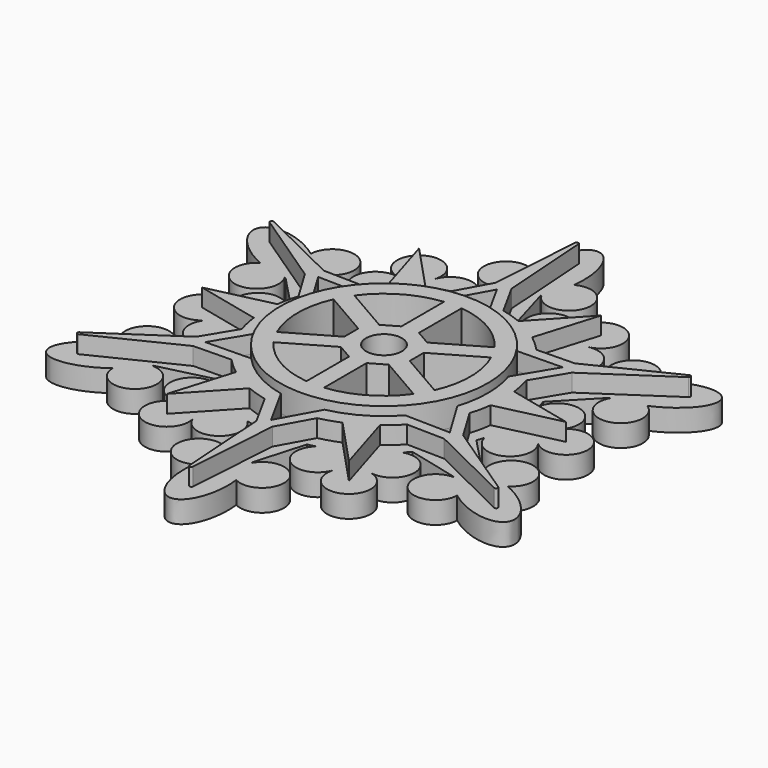
from build123d import *
from build123d import SkipClean  # not in build123d's __all__

# Parameters (mm, degrees)
F1_DEPTH      = 0.5
F3_DEPTH      = 0.4
F4_R          = 2.3683701977
F5_DEPTH      = 0.2
F5_DEPTH_BACK = 0.9
F6_R          = 0.4084956612
F7_DEPTH      = 1.1
F9_DEPTH      = 0.5


with BuildPart() as f1:
    # F0 (on Top) → F1 (new body)
    with BuildSketch(Plane.XY):
        with BuildLine():
            ThreePointArc((2.1292437706, 2.1379604716), (2.784209027, 2.5873993383), (2.1788959991, 3.1017639174))
            ThreePointArc((2.1788959991, 3.1017639174), (2.3229207895, 4.0234168295), (1.5967583495, 3.4378612461))
            ThreePointArc((1.5967583495, 3.4378612461), (0.8486490432, 3.704895416), (0.7869061954, 2.912959432))
            ThreePointArc((0.7869061954, 2.912959432), (0.6988064817, 2.9353404426), (0.6100725944, 2.9550576039))
            Line((0.6100725944, 2.9550576039), (0.2748547939, 4.1143940162))
            Line((0.2748547939, 4.1143940162), (0.2878654298, 4.1219057103))
            ThreePointArc((0.2878654298, 4.1219057103), (1.2019532573, 4.2356459456), (0.4832848134, 4.8118482237))
            add(Edge.make_bspline(
                [(0.4832848134, 4.8118482237), (0.6439857116, 6.079306826), (0, 6.079306826), (-0.6439857116, 6.079306826), (-0.4832848134, 4.8118482237)],
                knots=[4.4601826536, 4.4601826536, 4.4601826536, 6.2831853072, 6.2831853072, 8.1061879607, 8.1061879607, 8.1061879607], degree=2, weights=[1, 0.6125597551, 1, 0.6125597551, 1]))
            ThreePointArc((-0.4832848134, 4.8118482237), (-1.2019532573, 4.2356459456), (-0.2878654298, 4.1219057103))
            Line((-0.2878654298, 4.1219057103), (-0.2748547939, 4.1143940162))
            Line((-0.2748547939, 4.1143940162), (-0.6100725944, 2.9550576039))
            ThreePointArc((-0.6100725944, 2.9550576039), (-0.6988064817, 2.9353404426), (-0.7869061954, 2.912959432))
            ThreePointArc((-0.7869061954, 2.912959432), (-0.8486490432, 3.704895416), (-1.5967583495, 3.4378612461))
            ThreePointArc((-1.5967583495, 3.4378612461), (-2.3229207895, 4.0234168295), (-2.1788959991, 3.1017639174))
            ThreePointArc((-2.1788959991, 3.1017639174), (-2.784209027, 2.5873993383), (-2.1292437706, 2.1379604716))
            ThreePointArc((-2.1292437706, 2.1379604716), (-2.1926761512, 2.0728543867), (-2.2541186574, 2.0058671668))
            Line((-2.2541186574, 2.0058671668), (-3.4257423422, 2.2952282419))
            Line((-3.4257423422, 2.2952282419), (-3.4257423422, 2.3102516302))
            ThreePointArc((-3.4257423422, 2.3102516302), (-3.0672003617, 3.1587450278), (-3.9255403942, 2.8244610375))
            add(Edge.make_bspline(
                [(-3.9255403942, 2.8244610375), (-4.9428412929, 3.5973613989), (-5.2648341487, 3.039653413), (-5.5868270045, 2.4819454271), (-4.4088252076, 1.9873871862)],
                knots=[4.4601826536, 4.4601826536, 4.4601826536, 6.2831853072, 6.2831853072, 8.1061879607, 8.1061879607, 8.1061879607], degree=2, weights=[1, 0.6125597551, 1, 0.6125597551, 1]))
            ThreePointArc((-4.4088252076, 1.9873871862), (-4.269153619, 1.0769009178), (-3.713607772, 1.8116540801))
            Line((-3.713607772, 1.8116540801), (-3.7005971361, 1.8191657742))
            Line((-3.7005971361, 1.8191657742), (-2.8641912518, 0.9491904371))
            ThreePointArc((-2.8641912518, 0.9491904371), (-2.8914826329, 0.8624860559), (-2.916149966, 0.7749989604))
            ThreePointArc((-2.916149966, 0.7749989604), (-3.6328580702, 1.1174960777), (-3.7756543486, 0.3360973287))
            ThreePointArc((-3.7756543486, 0.3360973287), (-4.6458415791, 0), (-3.7756543486, -0.3360973287))
            ThreePointArc((-3.7756543486, -0.3360973287), (-3.6328580702, -1.1174960777), (-2.916149966, -0.7749989604))
            ThreePointArc((-2.916149966, -0.7749989604), (-2.8914826329, -0.8624860559), (-2.8641912518, -0.9491904371))
            Line((-2.8641912518, -0.9491904371), (-3.7005971361, -1.8191657742))
            Line((-3.7005971361, -1.8191657742), (-3.713607772, -1.8116540801))
            ThreePointArc((-3.713607772, -1.8116540801), (-4.269153619, -1.0769009178), (-4.4088252076, -1.9873871862))
            add(Edge.make_bspline(
                [(-4.4088252076, -1.9873871862), (-5.5868270045, -2.4819454271), (-5.2648341487, -3.039653413), (-4.9428412929, -3.5973613989), (-3.9255403942, -2.8244610375)],
                knots=[4.4601826536, 4.4601826536, 4.4601826536, 6.2831853072, 6.2831853072, 8.1061879607, 8.1061879607, 8.1061879607], degree=2, weights=[1, 0.6125597551, 1, 0.6125597551, 1]))
            ThreePointArc((-3.9255403942, -2.8244610375), (-3.0672003617, -3.1587450278), (-3.4257423422, -2.3102516302))
            Line((-3.4257423422, -2.3102516302), (-3.4257423422, -2.2952282419))
            Line((-3.4257423422, -2.2952282419), (-2.2541186574, -2.0058671668))
            ThreePointArc((-2.2541186574, -2.0058671668), (-2.1926761512, -2.0728543867), (-2.1292437706, -2.1379604716))
            ThreePointArc((-2.1292437706, -2.1379604716), (-2.784209027, -2.5873993383), (-2.1788959991, -3.1017639174))
            ThreePointArc((-2.1788959991, -3.1017639174), (-2.3229207895, -4.0234168295), (-1.5967583495, -3.4378612461))
            ThreePointArc((-1.5967583495, -3.4378612461), (-0.8486490432, -3.704895416), (-0.7869061954, -2.912959432))
            ThreePointArc((-0.7869061954, -2.912959432), (-0.6988064817, -2.9353404426), (-0.6100725944, -2.9550576039))
            Line((-0.6100725944, -2.9550576039), (-0.2748547939, -4.1143940162))
            Line((-0.2748547939, -4.1143940162), (-0.2878654298, -4.1219057103))
            ThreePointArc((-0.2878654298, -4.1219057103), (-1.2019532573, -4.2356459456), (-0.4832848134, -4.8118482237))
            add(Edge.make_bspline(
                [(-0.4832848134, -4.8118482237), (-0.6439857116, -6.079306826), (0, -6.079306826), (0.6439857116, -6.079306826), (0.4832848134, -4.8118482237)],
                knots=[4.4601826536, 4.4601826536, 4.4601826536, 6.2831853072, 6.2831853072, 8.1061879607, 8.1061879607, 8.1061879607], degree=2, weights=[1, 0.6125597551, 1, 0.6125597551, 1]))
            ThreePointArc((0.4832848134, -4.8118482237), (1.2019532573, -4.2356459456), (0.2878654298, -4.1219057103))
            Line((0.2878654298, -4.1219057103), (0.2748547939, -4.1143940162))
            Line((0.2748547939, -4.1143940162), (0.6100725944, -2.9550576039))
            ThreePointArc((0.6100725944, -2.9550576039), (0.6988064817, -2.9353404426), (0.7869061954, -2.912959432))
            ThreePointArc((0.7869061954, -2.912959432), (0.8486490432, -3.704895416), (1.5967583495, -3.4378612461))
            ThreePointArc((1.5967583495, -3.4378612461), (2.3229207895, -4.0234168295), (2.1788959991, -3.1017639174))
            ThreePointArc((2.1788959991, -3.1017639174), (2.784209027, -2.5873993383), (2.1292437706, -2.1379604716))
            ThreePointArc((2.1292437706, -2.1379604716), (2.1926761512, -2.0728543867), (2.2541186574, -2.0058671668))
            Line((2.2541186574, -2.0058671668), (3.4257423422, -2.2952282419))
            Line((3.4257423422, -2.2952282419), (3.4257423422, -2.3102516302))
            ThreePointArc((3.4257423422, -2.3102516302), (3.0672003617, -3.1587450278), (3.9255403942, -2.8244610375))
            add(Edge.make_bspline(
                [(3.9255403942, -2.8244610375), (4.9428412929, -3.5973613989), (5.2648341487, -3.039653413), (5.5868270045, -2.4819454271), (4.4088252076, -1.9873871862)],
                knots=[4.4601826536, 4.4601826536, 4.4601826536, 6.2831853072, 6.2831853072, 8.1061879607, 8.1061879607, 8.1061879607], degree=2, weights=[1, 0.6125597551, 1, 0.6125597551, 1]))
            ThreePointArc((4.4088252076, -1.9873871862), (4.269153619, -1.0769009178), (3.713607772, -1.8116540801))
            Line((3.713607772, -1.8116540801), (3.7005971361, -1.8191657742))
            Line((3.7005971361, -1.8191657742), (2.8641912518, -0.9491904371))
            ThreePointArc((2.8641912518, -0.9491904371), (2.8914826329, -0.8624860559), (2.916149966, -0.7749989604))
            ThreePointArc((2.916149966, -0.7749989604), (3.6328580702, -1.1174960777), (3.7756543486, -0.3360973287))
            ThreePointArc((3.7756543486, -0.3360973287), (4.6458415791, 0), (3.7756543486, 0.3360973287))
            ThreePointArc((3.7756543486, 0.3360973287), (3.6328580702, 1.1174960777), (2.916149966, 0.7749989604))
            ThreePointArc((2.916149966, 0.7749989604), (2.8914826329, 0.8624860559), (2.8641912518, 0.9491904371))
            Line((2.8641912518, 0.9491904371), (3.7005971361, 1.8191657742))
            Line((3.7005971361, 1.8191657742), (3.713607772, 1.8116540801))
            ThreePointArc((3.713607772, 1.8116540801), (4.269153619, 1.0769009178), (4.4088252076, 1.9873871862))
            add(Edge.make_bspline(
                [(4.4088252076, 1.9873871862), (5.5868270045, 2.4819454271), (5.2648341487, 3.039653413), (4.9428412929, 3.5973613989), (3.9255403942, 2.8244610375)],
                knots=[4.4601826536, 4.4601826536, 4.4601826536, 6.2831853072, 6.2831853072, 8.1061879607, 8.1061879607, 8.1061879607], degree=2, weights=[1, 0.6125597551, 1, 0.6125597551, 1]))
            ThreePointArc((3.9255403942, 2.8244610375), (3.0672003617, 3.1587450278), (3.4257423422, 2.3102516302))
            Line((3.4257423422, 2.3102516302), (3.4257423422, 2.2952282419))
            Line((3.4257423422, 2.2952282419), (2.2541186574, 2.0058671668))
            ThreePointArc((2.2541186574, 2.0058671668), (2.1926761512, 2.0728543867), (2.1292437706, 2.1379604716))
        make_face()
    extrude(amount=F1_DEPTH)

    # F2 (on face) → F3 (join)
    with BuildSketch(Plane.XY.offset(0.5)):
        with BuildLine():
            Line((-0.1806932342, 3.4074762445), (-0.597129254, 2.6519753366))
            ThreePointArc((-0.597129254, 2.6519753366), (-0.8306085867, 2.5883635578), (-1.0575056858, 2.5042400557))
            ThreePointArc((-1.0575056858, 2.5042400557), (-1.3591850989, 2.3541776481), (-1.6399826625, 2.1679468164))
            ThreePointArc((-1.6399826625, 2.1679468164), (-1.826284302, 2.0135099156), (-1.9981133847, 1.8431167716))
            Line((-1.9981133847, 1.8431167716), (-2.8606143735, 1.8602230533))
            Line((-2.8606143735, 1.8602230533), (-4.7338257783, 2.7791583452))
            ThreePointArc((-4.7338257783, 2.7791583452), (-4.7860838158, 2.7632467794), (-4.7737346173, 2.7100342085))
            Line((-4.7737346173, 2.7100342085), (-3.0413076076, 1.5472531912))
            Line((-3.0413076076, 1.5472531912), (-2.5952426387, 0.808858565))
            ThreePointArc((-2.5952426387, 0.808858565), (-2.6568928887, 0.5748536422), (-2.6974883483, 0.3362932393))
            ThreePointArc((-2.6974883483, 0.3362932393), (-2.7183701977, 0), (-2.6974883483, -0.3362932393))
            ThreePointArc((-2.6974883483, -0.3362932393), (-2.6568928887, -0.5748536422), (-2.5952426387, -0.808858565))
            Line((-2.5952426387, -0.808858565), (-3.0413076076, -1.5472531912))
            Line((-3.0413076076, -1.5472531912), (-4.7737346173, -2.7100342085))
            ThreePointArc((-4.7737346173, -2.7100342085), (-4.7860838158, -2.7632467794), (-4.7338257783, -2.7791583452))
            Line((-4.7338257783, -2.7791583452), (-2.8606143735, -1.8602230533))
            Line((-2.8606143735, -1.8602230533), (-1.9981133847, -1.8431167716))
            ThreePointArc((-1.9981133847, -1.8431167716), (-1.826284302, -2.0135099156), (-1.6399826625, -2.1679468164))
            ThreePointArc((-1.6399826625, -2.1679468164), (-1.3591850989, -2.3541776481), (-1.0575056858, -2.5042400557))
            ThreePointArc((-1.0575056858, -2.5042400557), (-0.8306085867, -2.5883635578), (-0.597129254, -2.6519753366))
            Line((-0.597129254, -2.6519753366), (-0.1806932342, -3.4074762445))
            Line((-0.1806932342, -3.4074762445), (-0.039908839, -5.4891925537))
            ThreePointArc((-0.039908839, -5.4891925537), (0, -5.5264935588), (0.039908839, -5.4891925537))
            Line((0.039908839, -5.4891925537), (0.1806932342, -3.4074762445))
            Line((0.1806932342, -3.4074762445), (0.597129254, -2.6519753366))
            ThreePointArc((0.597129254, -2.6519753366), (0.8306085867, -2.5883635578), (1.0575056858, -2.5042400557))
            ThreePointArc((1.0575056858, -2.5042400557), (1.3591850989, -2.3541776481), (1.6399826625, -2.1679468164))
            ThreePointArc((1.6399826625, -2.1679468164), (1.826284302, -2.0135099156), (1.9981133847, -1.8431167716))
            Line((1.9981133847, -1.8431167716), (2.8606143735, -1.8602230533))
            Line((2.8606143735, -1.8602230533), (4.7338257783, -2.7791583452))
            ThreePointArc((4.7338257783, -2.7791583452), (4.7860838158, -2.7632467794), (4.7737346173, -2.7100342085))
            Line((4.7737346173, -2.7100342085), (3.0413076076, -1.5472531912))
            Line((3.0413076076, -1.5472531912), (2.5952426387, -0.808858565))
            ThreePointArc((2.5952426387, -0.808858565), (2.6568928887, -0.5748536422), (2.6974883483, -0.3362932393))
            ThreePointArc((2.6974883483, -0.3362932393), (2.7183701977, 0), (2.6974883483, 0.3362932393))
            ThreePointArc((2.6974883483, 0.3362932393), (2.6568928887, 0.5748536422), (2.5952426387, 0.808858565))
            Line((2.5952426387, 0.808858565), (3.0413076076, 1.5472531912))
            Line((3.0413076076, 1.5472531912), (4.7737346173, 2.7100342085))
            ThreePointArc((4.7737346173, 2.7100342085), (4.7860838158, 2.7632467794), (4.7338257783, 2.7791583452))
            Line((4.7338257783, 2.7791583452), (2.8606143735, 1.8602230533))
            Line((2.8606143735, 1.8602230533), (1.9981133847, 1.8431167716))
            ThreePointArc((1.9981133847, 1.8431167716), (1.826284302, 2.0135099156), (1.6399826625, 2.1679468164))
            ThreePointArc((1.6399826625, 2.1679468164), (1.3591850989, 2.3541776481), (1.0575056858, 2.5042400557))
            ThreePointArc((1.0575056858, 2.5042400557), (0.8306085867, 2.5883635578), (0.597129254, 2.6519753366))
            Line((0.597129254, 2.6519753366), (0.1806932342, 3.4074762445))
            Line((0.1806932342, 3.4074762445), (0.039908839, 5.4891925537))
            ThreePointArc((0.039908839, 5.4891925537), (0, 5.5264935588), (-0.039908839, 5.4891925537))
            Line((-0.039908839, 5.4891925537), (-0.1806932342, 3.4074762445))
        make_face()
        Polygon((-2.1979116775, -0.6346252141), (-1.6485573961, -1.5861347409), (-2.786351891, -1.6087010143), align=None, mode=Mode.SUBTRACT)
        Polygon((-0.5493542814, -2.220759955), (0.5493542814, -2.220759955), (0, -3.2174020287), align=None, mode=Mode.SUBTRACT)
        Polygon((1.6485573961, -1.5861347409), (2.1979116775, -0.6346252141), (2.786351891, -1.6087010143), align=None, mode=Mode.SUBTRACT)
        Polygon((-1.6485573961, 1.5861347409), (-2.1979116775, 0.6346252141), (-2.786351891, 1.6087010143), align=None, mode=Mode.SUBTRACT)
        Polygon((2.1979116775, 0.6346252141), (1.6485573961, 1.5861347409), (2.786351891, 1.6087010143), align=None, mode=Mode.SUBTRACT)
        Polygon((-0.5493542814, 2.220759955), (0, 3.2174020287), (0.5493542814, 2.220759955), align=None, mode=Mode.SUBTRACT)
        with BuildLine():
            ThreePointArc((-1.6399826625, 2.1679468164), (-1.3591850989, 2.3541776481), (-1.0575056858, 2.5042400557))
            Line((-1.0575056858, 2.5042400557), (-2.0729207895, 3.5904041276))
            Line((-2.0729207895, 3.5904041276), (-1.6399826625, 2.1679468164))
        make_face()
        with BuildLine():
            Line((2.0729207895, 3.5904041276), (1.0575056858, 2.5042400557))
            ThreePointArc((1.0575056858, 2.5042400557), (1.3591850989, 2.3541776481), (1.6399826625, 2.1679468164))
            Line((1.6399826625, 2.1679468164), (2.0729207895, 3.5904041276))
        make_face()
        with BuildLine():
            ThreePointArc((-2.6974883483, -0.3362932393), (-2.7183701977, 0), (-2.6974883483, 0.3362932393))
            Line((-2.6974883483, 0.3362932393), (-4.1458415791, 0))
            Line((-4.1458415791, 0), (-2.6974883483, -0.3362932393))
        make_face()
        with BuildLine():
            Line((4.1458415791, 0), (2.6974883483, 0.3362932393))
            ThreePointArc((2.6974883483, 0.3362932393), (2.7183701977, 0), (2.6974883483, -0.3362932393))
            Line((2.6974883483, -0.3362932393), (4.1458415791, 0))
        make_face()
        with BuildLine():
            ThreePointArc((-1.0575056858, -2.5042400557), (-1.3591850989, -2.3541776481), (-1.6399826625, -2.1679468164))
            Line((-1.6399826625, -2.1679468164), (-2.0729207895, -3.5904041276))
            Line((-2.0729207895, -3.5904041276), (-1.0575056858, -2.5042400557))
        make_face()
        with BuildLine():
            Line((2.0729207895, -3.5904041276), (1.6399826625, -2.1679468164))
            ThreePointArc((1.6399826625, -2.1679468164), (1.3591850989, -2.3541776481), (1.0575056858, -2.5042400557))
            Line((1.0575056858, -2.5042400557), (2.0729207895, -3.5904041276))
        make_face()
    extrude(amount=F3_DEPTH)

    # F4 (on face) → F5 (join, two sides)
    with BuildSketch(Plane.XY.offset(0.9)) as f5_sk:
        Circle(F4_R)
    extrude(amount=F5_DEPTH)
    extrude(f5_sk.sketch, amount=-F5_DEPTH_BACK)

    # F6 (on face) → F7 (cut, through all)
    with BuildSketch(Plane.XY.offset(1.1)):
        with BuildLine():
            Line((-0.2, 0.7464101615), (-0.2, 1.9581831465))
            ThreePointArc((-0.2, 1.9581831465), (-0.9841850989, 1.7046585953), (-1.5958363501, 1.152296654))
            Line((-1.5958363501, 1.152296654), (-0.5464101615, 0.5464101615))
            Line((-0.5464101615, 0.5464101615), (-0.2, 0.7464101615))
        make_face()
        with BuildLine():
            Line((-0.7464101615, 0.2), (-1.7958363501, 0.8058864925))
            ThreePointArc((-1.7958363501, 0.8058864925), (-1.9683701977, 0), (-1.7958363501, -0.8058864925))
            Line((-1.7958363501, -0.8058864925), (-0.7464101615, -0.2))
            Line((-0.7464101615, -0.2), (-0.7464101615, 0.2))
        make_face()
        with BuildLine():
            Line((-0.5464101615, -0.5464101615), (-1.5958363501, -1.152296654))
            ThreePointArc((-1.5958363501, -1.152296654), (-0.9841850989, -1.7046585953), (-0.2, -1.9581831465))
            Line((-0.2, -1.9581831465), (-0.2, -0.7464101615))
            Line((-0.2, -0.7464101615), (-0.5464101615, -0.5464101615))
        make_face()
        with BuildLine():
            Line((0.2, -0.7464101615), (0.2, -1.9581831465))
            ThreePointArc((0.2, -1.9581831465), (0.9841850989, -1.7046585953), (1.5958363501, -1.152296654))
            Line((1.5958363501, -1.152296654), (0.5464101615, -0.5464101615))
            Line((0.5464101615, -0.5464101615), (0.2, -0.7464101615))
        make_face()
        with BuildLine():
            Line((0.7464101615, -0.2), (1.7958363501, -0.8058864925))
            ThreePointArc((1.7958363501, -0.8058864925), (1.9683701977, 0), (1.7958363501, 0.8058864925))
            Line((1.7958363501, 0.8058864925), (0.7464101615, 0.2))
            Line((0.7464101615, 0.2), (0.7464101615, -0.2))
        make_face()
        with BuildLine():
            Line((0.5464101615, 0.5464101615), (1.5958363501, 1.152296654))
            ThreePointArc((1.5958363501, 1.152296654), (0.9841850989, 1.7046585953), (0.2, 1.9581831465))
            Line((0.2, 1.9581831465), (0.2, 0.7464101615))
            Line((0.2, 0.7464101615), (0.5464101615, 0.5464101615))
        make_face()
        Circle(F6_R)
    extrude(amount=-F7_DEPTH, mode=Mode.SUBTRACT)

    # F8 (on face) → F9 (cut, through all)
    with BuildSketch(Plane.XY.offset(0.5)):
        with BuildLine():
            Line((0.4970661396, 2.3156214385), (0, 3.2174020287))
            Line((0, 3.2174020287), (-0.4970661396, 2.3156214385))
            ThreePointArc((-0.4970661396, 2.3156214385), (0, 2.3683701977), (0.4970661396, 2.3156214385))
        make_face()
        with BuildLine():
            ThreePointArc((-2.2539200611, 0.727338815), (-2.0510687568, 1.1841850989), (-1.7568539215, 1.5882826235))
            Line((-1.7568539215, 1.5882826235), (-2.786351891, 1.6087010143))
            Line((-2.786351891, 1.6087010143), (-2.2539200611, 0.727338815))
        make_face()
        with BuildLine():
            Line((2.786351891, 1.6087010143), (1.7568539215, 1.5882826235))
            ThreePointArc((1.7568539215, 1.5882826235), (2.0510687568, 1.1841850989), (2.2539200611, 0.727338815))
            Line((2.2539200611, 0.727338815), (2.786351891, 1.6087010143))
        make_face()
        with BuildLine():
            Line((2.786351891, -1.6087010143), (2.2539200611, -0.727338815))
            ThreePointArc((2.2539200611, -0.727338815), (2.0510687568, -1.1841850989), (1.7568539215, -1.5882826235))
            Line((1.7568539215, -1.5882826235), (2.786351891, -1.6087010143))
        make_face()
        with BuildLine():
            Line((0, -3.2174020287), (0.4970661396, -2.3156214385))
            ThreePointArc((0.4970661396, -2.3156214385), (0, -2.3683701977), (-0.4970661396, -2.3156214385))
            Line((-0.4970661396, -2.3156214385), (0, -3.2174020287))
        make_face()
        with BuildLine():
            Line((-2.786351891, -1.6087010143), (-1.7568539215, -1.5882826235))
            ThreePointArc((-1.7568539215, -1.5882826235), (-2.0510687568, -1.1841850989), (-2.2539200611, -0.727338815))
            Line((-2.2539200611, -0.727338815), (-2.786351891, -1.6087010143))
        make_face()
    with SkipClean():  # cleaning this boolean's faces spoils the solid; the shape is the same uncleaned
        extrude(amount=-F9_DEPTH, mode=Mode.SUBTRACT)


solid = f1.part
